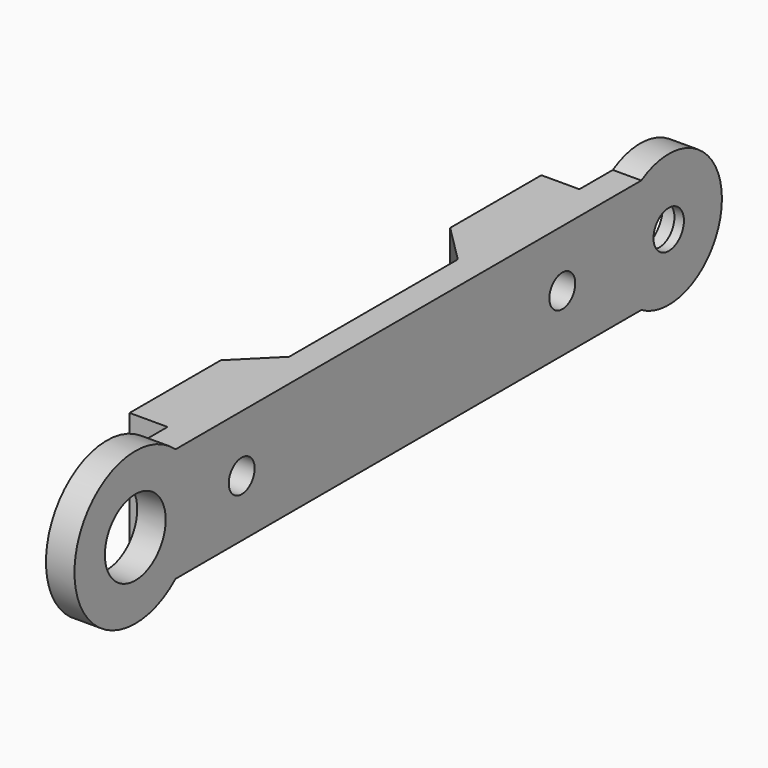
from build123d import *

# Parameters (mm, degrees)
F1_DEPTH = 9.525
F2_R     = 5.55625
F2_R_2   = 6.35
F3_DEPTH = 2.38125
F4_R     = 3.175
F4_R_2   = 1.35255
F4_R_3   = 1.5875
F5_DEPTH = 5.55625
F6_R     = 2.38125
F7_DEPTH = 1.5875
F8_SIZE  = 3.17499


# Not quite as in the source:
# - a fillet or chamfer is up to 0.001 mm smaller than in the source, because OpenCascade refuses the exact size


with BuildPart() as f1:
    # F0 (on Top) → F1 (new body)
    with BuildSketch(Plane.XY):
        Polygon((0, 0), (0, 55.7060608), (-2.38125, 55.7060608), (-2.38125, 49.3560608), (-5.55625, 49.3560608), (-5.55625, 39.8310608), (-2.38125, 39.8310608), (-2.38125, 15.875), (-5.55625, 15.875), (-5.55625, 6.35), (-2.38125, 6.35), (-2.38125, 0), align=None)
    extrude(amount=F1_DEPTH)

    # F2 (on face) → F3 (join, through all)
    with BuildSketch(Plane(origin=(-2.38125, 0, 0), x_dir=(0, -1, 0), z_dir=(-1, 0, 0))):
        with Locations((-55.7060608, 4.7625)):
            Circle(F2_R)
        with Locations((0, 4.7625)):
            Circle(F2_R_2)
    extrude(amount=-F3_DEPTH)

    # F4 (on face) → F5 (cut, through all)
    with BuildSketch(Plane.YZ):
        with Locations((0, 4.7625)):
            Circle(F4_R)
        with Locations((11.1125, 4.7625)):
            Circle(F4_R_2)
        with Locations((44.5935608, 4.7625)):
            Circle(F4_R_2)
        with Locations((55.7060608001, 4.7625)):
            Circle(F4_R_3)
    extrude(amount=-F5_DEPTH, mode=Mode.SUBTRACT)

    # F6 (on face) → F7 (cut)
    with BuildSketch(Plane(origin=(-2.38125, 0, 0), x_dir=(0, -1, 0), z_dir=(-1, 0, 0))):
        with Locations((-55.7060608, 4.7625)):
            Circle(F6_R)
    extrude(amount=-F7_DEPTH, mode=Mode.SUBTRACT)

    # F8 (size 3.175 in the source; OpenCascade refuses exactly that, so slightly less here)
    f8_edges = [f1.edges().sort_by_distance(p)[0] for p in [
        (-2.38125, 39.831061, 4.7625),
        (-2.38125, 15.875, 4.7625),
    ]]
    chamfer(f8_edges, length=F8_SIZE)


solid = f1.part
